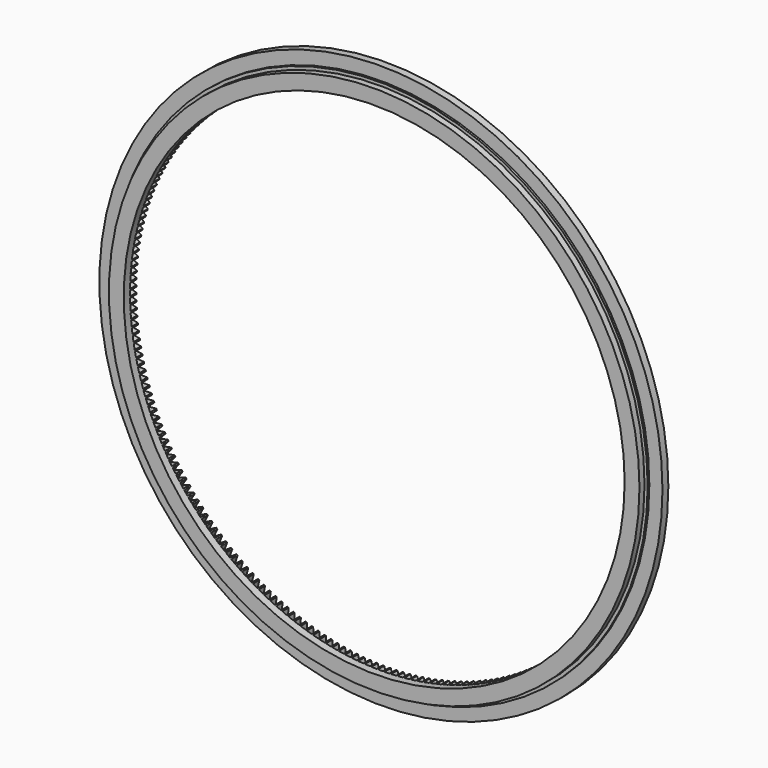
from build123d import *

# Parameters (mm, degrees)
F0_R            = 67
F0_R_2          = 59.6
F1_DEPTH        = 1.875
F2_R            = 63.875
F2_R_2          = 63.125
F3_DEPTH        = 1.5
F4_DEPTH        = 2
F6_DEPTH        = 7.5
F6_COPIES_COUNT = 240


# Not quite as in the source:
# - a feature of the source that left no trace in its solid (it failed there, or was rolled back) is left out
# - a pattern or mirror of a feature is missing from the dataset's text; its kind, count and spacing are read off the source's solid
# - a feature names something its author has since deleted; it is built from what else it names


with BuildPart() as f1:
    # F0 (on Front) → F1 (new body, symmetric)
    with BuildSketch(Plane.XZ):
        Circle(F0_R)
        Circle(F0_R_2, mode=Mode.SUBTRACT)
    extrude(amount=F1_DEPTH, both=True)

    # F2 (on face) → F3 (cut)
    with BuildSketch(Plane.XZ.offset(1.875)):
        Circle(F2_R)
        Circle(F2_R_2, mode=Mode.SUBTRACT)
    extrude(amount=-F3_DEPTH, mode=Mode.SUBTRACT)

    # F4 (cut): a face of the model
    f4_faces = [f1.faces().sort_by_distance(p)[0] for p in [
        (-65.1049538264, -1.875, 0),
    ]]
    extrude(f4_faces, amount=-F4_DEPTH, mode=Mode.SUBTRACT)

    # F5 (on Front) → F6 (cut)
    with BuildSketch(Plane.XZ):
        with BuildLine():
            Line((-59.4, 0.675), (-60.9998154245, 0.1500605638))
            ThreePointArc((-60.9998154245, 0.1500605638), (-60.9999538561, 0.0750303387), (-61, 0))
            Line((-61, 0), (-59.4, 0))
            Line((-59.4, 0), (-59.4, 0.675))
        make_face()
        with BuildLine():
            ThreePointArc((-61, 0), (-60.9999538561, -0.0750303387), (-60.9998154245, -0.1500605638))
            Line((-60.9998154245, -0.1500605638), (-59.4, -0.675))
            Line((-59.4, -0.675), (-59.4, 0))
            Line((-59.4, 0), (-61, 0))
        make_face()
    f6 = extrude(amount=-F6_DEPTH, mode=Mode.SUBTRACT)

    # F6_copies: F6 ×240 about axis
    f6_copies_axis = Axis((0, 0, 0), (0, 1, 0))
    for i in range(1, F6_COPIES_COUNT):
        add(f6.rotate(f6_copies_axis, i * 360 / F6_COPIES_COUNT), mode=Mode.SUBTRACT)


solid = f1.part
